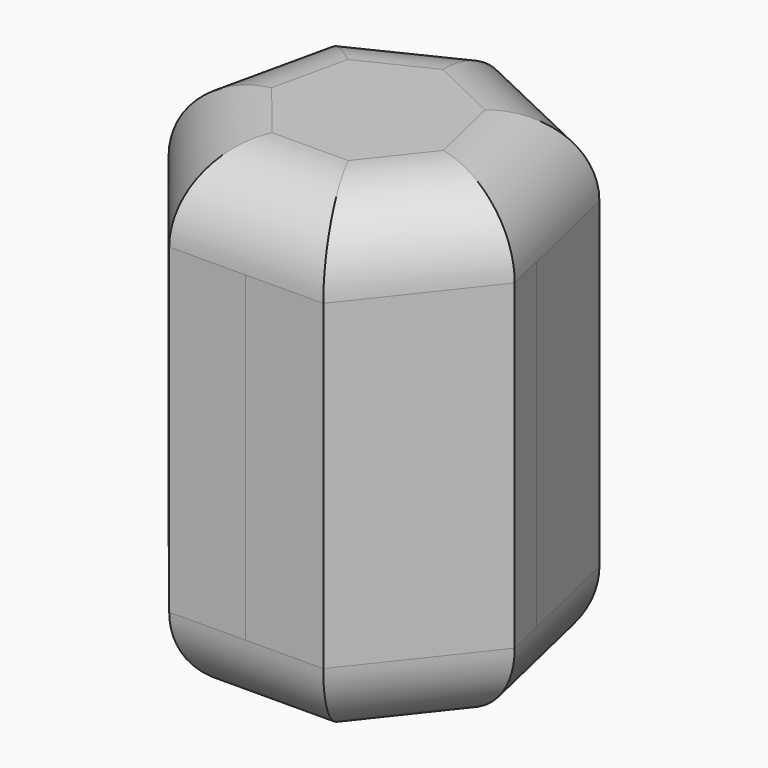
from build123d import *

# Parameters (mm, degrees)
F1_DEPTH     = 76.2
F2_T1_DEPTH  = 175.4963381321
F2_T3_DEPTH  = 175.4963381321
F2_T5_DEPTH  = 175.4963381321
F2_T7_DEPTH  = 175.4963381321
F2_T9_DEPTH  = 175.4963381321
F2_T11_DEPTH = 175.4963381321
F2_T13_DEPTH = 175.4963381321


# Not quite as in the source:
# - a fillet or chamfer that OpenCascade refuses, or shapes differently, is made with other operations: its cross-section is extruded or revolved along the edge and cut away or added


with BuildPart() as f1:
    # F0 (on Top) → F1 (new body, symmetric)
    with BuildSketch(Plane.XY):
        Polygon((0, 0), (0, 55.7593321666), (-0.2656214809, 55.8856970104), (-43.8588096269, 34.6364909196), align=None)
        Polygon((0, 0), (43.5275850579, 35.051833392), (0, 55.7593321666), align=None)
        Polygon((51.7034059885, 0), (43.5275850579, 35.051833392), (0, 0), align=None)
        Polygon((24.487211867, -50.2360243261), (54.5436322472, -12.1767756978), (0, 0), align=None)
        Polygon((0, -50.3524106258), (0, 0), (-24.0085784972, -50.4665220087), align=None)
        Polygon((24.487211867, -50.2360243261), (0, 0), (0, -50.3524106258), align=None)
        Polygon((-24.0085784972, -50.4665220087), (0, 0), (-54.4254195672, -12.6946992894), align=None)
        Polygon((-51.5913489447, 0), (0, 0), (-43.8588096269, 34.6364909196), align=None)
        Polygon((-54.4254195672, -12.6946992894), (0, 0), (-51.5913489447, 0), align=None)
        Polygon((0, 0), (54.5436322472, -12.1767756978), (51.7034059885, 0), align=None)
    extrude(amount=F1_DEPTH, both=True)

    # F2: fillet of radius 25.4 on 14 edges, made by hand

    # F2_s2 → F2_t1 (cut)
    with BuildSketch(Plane(origin=(78.8765212158, 38.447829267, 0), x_dir=(0, 0, 1), z_dir=(-0.8988964904, -0.4381610429, 0))):
        with BuildLine():
            ThreePointArc((-50.8, 50.3518418934), (-68.7605122421, 42.9123541355), (-76.2, 24.9518418934))
            Line((-76.2, 24.9518418934), (-76.2, 50.3518418934))
            Line((-76.2, 50.3518418934), (-50.8, 50.3518418934))
        make_face()
        with BuildLine():
            ThreePointArc((50.8, 50.3518418934), (68.7605122421, 42.9123541355), (76.2, 24.9518418934))
            Line((76.2, 24.9518418934), (76.2, 50.3518418934))
            Line((76.2, 50.3518418934), (50.8, 50.3518418934))
        make_face()
    extrude(amount=F2_T1_DEPTH, mode=Mode.SUBTRACT)

    # F2_s4 → F2_t3 (cut)
    with BuildSketch(Plane(origin=(19.1189832306, 85.6399769656, 0), x_dir=(0, 0, 1), z_dir=(-0.217884697, -0.9759745175, 0))):
        with BuildLine():
            ThreePointArc((-50.8, 50.3518418934), (-68.7605122421, 42.9123541355), (-76.2, 24.9518418934))
            Line((-76.2, 24.9518418934), (-76.2, 50.3518418934))
            Line((-76.2, 50.3518418934), (-50.8, 50.3518418934))
        make_face()
        with BuildLine():
            ThreePointArc((76.2, 24.9518418934), (68.7605122421, 42.9123541355), (50.8, 50.3518418934))
            Line((50.8, 50.3518418934), (76.2, 50.3518418934))
            Line((76.2, 50.3518418934), (76.2, 24.9518418934))
        make_face()
    extrude(amount=F2_T3_DEPTH, mode=Mode.SUBTRACT)

    # F2_s6 → F2_t5 (cut)
    with BuildSketch(Plane(origin=(-55.0355390834, 68.343475272, 0), x_dir=(0, 0, 1), z_dir=(0.6271987173, -0.7788592742, 0))):
        with BuildLine():
            ThreePointArc((-50.8, 50.3518418934), (-68.7605122421, 42.9123541355), (-76.2, 24.9518418934))
            Line((-76.2, 24.9518418934), (-76.2, 50.3518418934))
            Line((-76.2, 50.3518418934), (-50.8, 50.3518418934))
        make_face()
        with BuildLine():
            ThreePointArc((50.8, 50.3518418934), (68.7605122421, 42.9123541355), (76.2, 24.9518418934))
            Line((76.2, 24.9518418934), (76.2, 50.3518418934))
            Line((76.2, 50.3518418934), (50.8, 50.3518418934))
        make_face()
    extrude(amount=F2_T5_DEPTH, mode=Mode.SUBTRACT)

    # F2_s8 → F2_t7 (cut)
    with BuildSketch(Plane(origin=(-87.7471779472, -0.4170572543, 0), x_dir=(0, 0, 1), z_dir=(0.999988705, 0.0047528884, 0))):
        with BuildLine():
            ThreePointArc((-50.8, 50.3518418934), (-68.7605122421, 42.9123541355), (-76.2, 24.9518418934))
            Line((-76.2, 24.9518418934), (-76.2, 50.3518418934))
            Line((-76.2, 50.3518418934), (-50.8, 50.3518418934))
        make_face()
        with BuildLine():
            ThreePointArc((50.8, 50.3518418934), (68.7605122421, 42.9123541355), (76.2, 24.9518418934))
            Line((76.2, 24.9518418934), (76.2, 50.3518418934))
            Line((76.2, 50.3518418934), (50.8, 50.3518418934))
        make_face()
    extrude(amount=F2_T7_DEPTH, mode=Mode.SUBTRACT)

    # F2_s10 → F2_t9 (cut)
    with BuildSketch(Plane(origin=(-54.3834021005, -68.8635371617, 0), x_dir=(0, 0, 1), z_dir=(0.6197668017, 0.7847860291, 0))):
        with BuildLine():
            ThreePointArc((-50.8, 50.3518418934), (-68.7605122421, 42.9123541355), (-76.2, 24.9518418934))
            Line((-76.2, 24.9518418934), (-76.2, 50.3518418934))
            Line((-76.2, 50.3518418934), (-50.8, 50.3518418934))
        make_face()
        with BuildLine():
            ThreePointArc((50.8, 50.3518418934), (68.7605122421, 42.9123541355), (76.2, 24.9518418934))
            Line((76.2, 24.9518418934), (76.2, 50.3518418934))
            Line((76.2, 50.3518418934), (50.8, 50.3518418934))
        make_face()
    extrude(amount=F2_T9_DEPTH, mode=Mode.SUBTRACT)

    # F2_s12 → F2_t11 (cut)
    with BuildSketch(Plane(origin=(19.932184747, -85.4543690261, 0), x_dir=(0, 0, 1), z_dir=(-0.2271521441, 0.9738592832, 0))):
        with BuildLine():
            ThreePointArc((-50.8, 50.3518418934), (-68.7605122421, 42.9123541355), (-76.2, 24.9518418934))
            Line((-76.2, 24.9518418934), (-76.2, 50.3518418934))
            Line((-76.2, 50.3518418934), (-50.8, 50.3518418934))
        make_face()
        with BuildLine():
            ThreePointArc((50.8, 50.3518418934), (68.7605122421, 42.9123541355), (76.2, 24.9518418934))
            Line((76.2, 24.9518418934), (76.2, 50.3518418934))
            Line((76.2, 50.3518418934), (50.8, 50.3518418934))
        make_face()
    extrude(amount=F2_T11_DEPTH, mode=Mode.SUBTRACT)

    # F2_s14 → F2_t13 (cut)
    with BuildSketch(Plane(origin=(79.2384299376, -37.6963180625, 0), x_dir=(0, 0, 1), z_dir=(-0.9030208924, 0.4295966339, 0))):
        with BuildLine():
            ThreePointArc((-50.8, 50.3518418934), (-68.7605122421, 42.9123541355), (-76.2, 24.9518418934))
            Line((-76.2, 24.9518418934), (-76.2, 50.3518418934))
            Line((-76.2, 50.3518418934), (-50.8, 50.3518418934))
        make_face()
        with BuildLine():
            ThreePointArc((50.8, 50.3518418934), (68.7605122421, 42.9123541355), (76.2, 24.9518418934))
            Line((76.2, 24.9518418934), (76.2, 50.3518418934))
            Line((76.2, 50.3518418934), (50.8, 50.3518418934))
        make_face()
    extrude(amount=F2_T13_DEPTH, mode=Mode.SUBTRACT)


solid = f1.part
